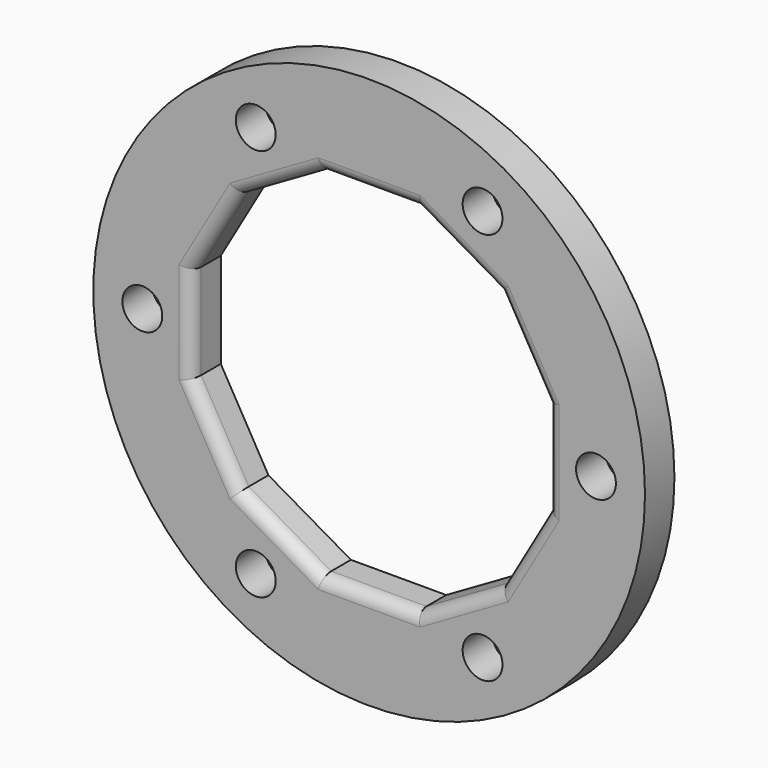
from build123d import *

# Parameters (mm, degrees)
F0_R            = 45
F1_DEPTH        = 3
F2_R            = 2
F3_R            = 3.25
F4_DEPTH        = 12.5
F4_COPIES_COUNT = 6


# Not quite as in the source:
# - a pattern or mirror of a feature is missing from the dataset's text; its kind, count and spacing are read off the source's solid


with BuildPart() as f1:
    # F0 (on Front) → F1 (new body, symmetric)
    with BuildSketch(Plane.XZ):
        Circle(F0_R)
        Polygon((-21.2294734195, 21.2294734195), (-7.7705265805, 29), (7.7705265805, 29), (21.2294734195, 21.2294734195), (29, 7.7705265805), (29, -7.7705265805), (21.2294734195, -21.2294734195), (7.7705265805, -29), (-7.7705265805, -29), (-21.2294734195, -21.2294734195), (-29, -7.7705265805), (-29, 7.7705265805), align=None, mode=Mode.SUBTRACT)
    extrude(amount=F1_DEPTH, both=True)

    # F2
    f2_edges = [f1.edges().sort_by_distance(p)[0] for p in [
        (-14.5, -3, 25.114737),
        (0, -3, 29),
        (14.5, -3, 25.114737),
        (25.114737, -3, 14.5),
        (29, -3, 0),
        (25.114737, -3, -14.5),
        (14.5, -3, -25.114737),
        (0, -3, -29),
        (-14.5, -3, -25.114737),
        (-25.114737, -3, -14.5),
        (-29, -3, 0),
        (-25.114737, -3, 14.5),
    ]]
    fillet(f2_edges, radius=F2_R)

    # F3 (on Front) → F4 (cut, symmetric)
    with BuildSketch(Plane.XZ):
        with Locations((37, 0)):
            Circle(F3_R)
    f4 = extrude(amount=F4_DEPTH, both=True, mode=Mode.SUBTRACT)

    # F4_copies: F4 ×6 about axis
    f4_copies_axis = Axis((0, 0, 0), (0, 1, 0))
    for i in range(1, F4_COPIES_COUNT):
        add(f4.rotate(f4_copies_axis, i * 360 / F4_COPIES_COUNT), mode=Mode.SUBTRACT)


solid = f1.part
